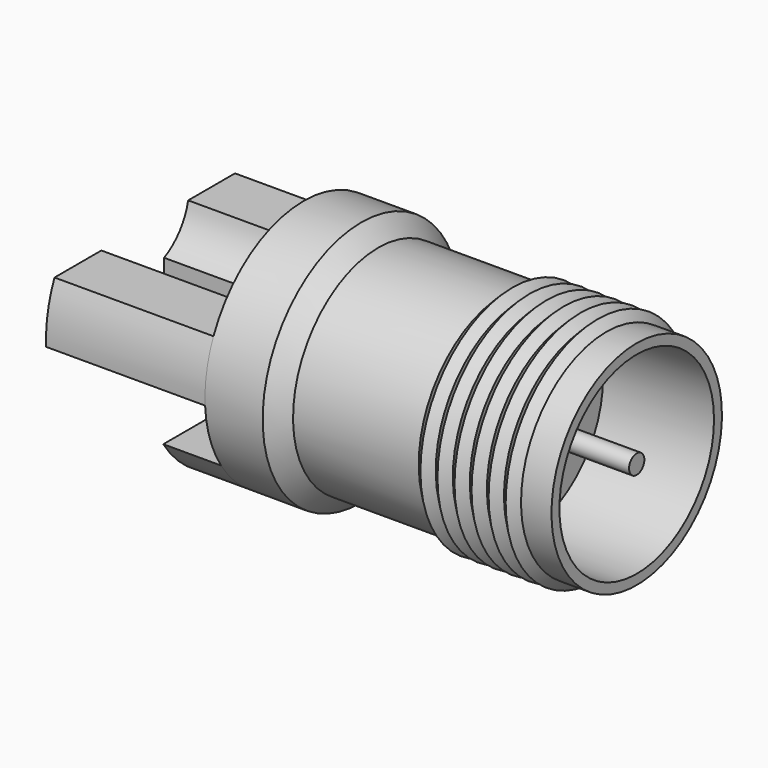
from build123d import *

# Parameters (mm, degrees)
F2_R     = 2.7634205328
F2_R_2   = 0.2730680528
F3_DEPTH = 3.175
F4_R     = 0.1905
F5_DEPTH = 1.016
F7_DEPTH = 1.651
F9_DEPTH = 4.5466


# Not quite as in the source:
# - after a boolean that leaves OpenCascade's solid faulty, fix() repairs it


with BuildPart() as f1:
    # F0 (on Front) → F1 (revolve)
    with BuildSketch(Plane.XZ):
        Polygon((0, 3.5306), (0, 0), (9.525, 0), (9.525, 3.048), (8.6543986211, 3.048), (8.4105280196, 3.2918706015), (8.1666574181, 3.048), (7.9227868167, 3.2918706015), (7.6789162152, 3.048), (7.4350456137, 3.2918706015), (7.1911750122, 3.048), (6.9473044108, 3.2918706015), (6.7034338093, 3.048), (6.4595632078, 3.2918706015), (6.2156926063, 3.048), (5.9718220049, 3.2918706015), (5.7279514034, 3.048), (2.1336, 3.048), (1.651, 3.5306), align=None)
    revolve(axis=Axis((4.7625, 0, 0), (1, 0, 0)))

    # F2 (on face) → F3 (cut)
    with BuildSketch(Plane.YZ.offset(9.525)):
        Circle(F2_R)
        Circle(F2_R_2, mode=Mode.SUBTRACT)
    extrude(amount=-F3_DEPTH, mode=Mode.SUBTRACT)

    # F4 (on face) → F5 (join)
    with BuildSketch(Plane(origin=(0, 0, 0), x_dir=(0, -1, 0), z_dir=(-1, 0, 0))):
        Circle(F4_R)
    extrude(amount=F5_DEPTH)

    # F6 (on face) → F7 (join)
    with BuildSketch(Plane(origin=(0, 0, 0), x_dir=(0, -1, 0), z_dir=(-1, 0, 0))):
        with BuildLine():
            ThreePointArc((-2.9561279066, -1.9304), (0, -3.5306), (2.9561279066, -1.9304))
            Line((2.9561279066, -1.9304), (-2.9561279066, -1.9304))
        make_face()
    extrude(amount=F7_DEPTH)

    add(f1.part.fix(), mode=Mode.REPLACE)

    # F8 (on face) → F9 (join)
    with BuildSketch(Plane(origin=(0, 0, 0), x_dir=(0, -1, 0), z_dir=(-1, 0, 0))):
        with BuildLine():
            Line((-1.5521158375, 1.4343592338), (-3.226104454, 1.4343592338))
            ThreePointArc((-3.226104454, 1.4343592338), (-3.4721660307, 0.6396869664), (-3.5254568654, -0.1905))
            Line((-3.5254568654, -0.1905), (-0.6920051213, -0.1905))
            Line((-0.6920051213, -0.1905), (-0.6920051213, 0.3389294034))
            ThreePointArc((-0.6920051213, 0.3389294034), (-1.2486037593, 0.7872849365), (-1.5521158375, 1.4343592338))
        make_face()
        with BuildLine():
            Line((0.6756495639, -0.1905), (3.5254568654, -0.1905))
            ThreePointArc((3.5254568654, -0.1905), (3.4721660307, 0.6396869664), (3.226104454, 1.4343592338))
            Line((3.226104454, 1.4343592338), (1.5521158375, 1.4343592338))
            ThreePointArc((1.5521158375, 1.4343592338), (1.2429873115, 0.7801737537), (0.6756495639, 0.3311225672))
            Line((0.6756495639, 0.3311225672), (0.6756495639, -0.1905))
        make_face()
    extrude(amount=F9_DEPTH)


solid = f1.part
